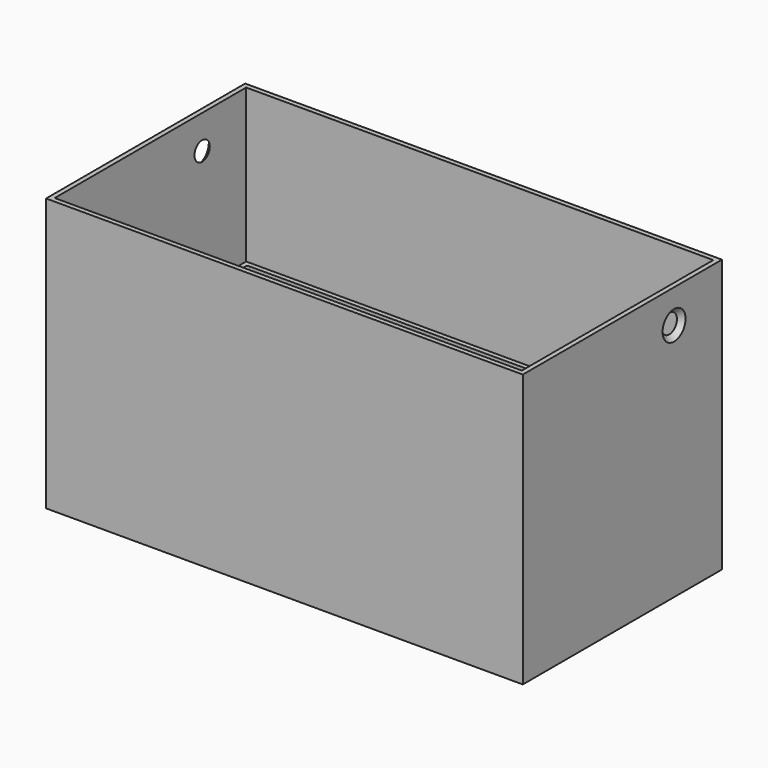
from build123d import *

# Parameters (mm, degrees)
F1_W          = 95.6
F1_H          = 48
F1_R          = 3
F1_R_2        = 1.75
F2_DEPTH      = 1.5
F1_W_2        = 97.6
F1_H_2        = 50
F3_DEPTH      = 25
F1_W_3        = 99.6
F1_H_3        = 52
F4_DEPTH      = 57
F5_R          = 2
F6_DEPTH      = 49.801
F6_DEPTH_BACK = 49.801
F7_SIZE       = 0.99999
F8_R          = 0.5


# Not quite as in the source:
# - a fillet or chamfer is up to 0.001 mm smaller than in the source, because OpenCascade refuses the exact size


with BuildPart() as f2:
    # F1 (on Top) → F2 (new body)
    with BuildSketch(Plane.XY):
        Rectangle(F1_W, F1_H)
        with Locations((-34.0166666667, 0)):
            Circle(F1_R, mode=Mode.SUBTRACT)
        with Locations((-20.2333333333, 0)):
            Circle(F1_R, mode=Mode.SUBTRACT)
        with Locations((-6.45, 0)):
            Circle(F1_R_2, mode=Mode.SUBTRACT)
        Polygon((-2.2, -13.3), (-2.2, 13.3), (35, 13.3), (40.3, 8), (40.3, -8), (35, -13.3), align=None, mode=Mode.SUBTRACT)
        with Locations((44.55, 0)):
            Circle(F1_R_2, mode=Mode.SUBTRACT)
    extrude(amount=F2_DEPTH)

    # F1 (on Top) → F3 (join)
    with BuildSketch(Plane.XY):
        Rectangle(F1_W_2, F1_H_2)
        Rectangle(F1_W, F1_H, mode=Mode.SUBTRACT)
    extrude(amount=F3_DEPTH)

    # F1 (on Top) → F4 (join)
    with BuildSketch(Plane.XY):
        Rectangle(F1_W_3, F1_H_3)
        Rectangle(F1_W_2, F1_H_2, mode=Mode.SUBTRACT)
    extrude(amount=F4_DEPTH)

    # F5 (on Right) → F6 (cut, two sides)
    with BuildSketch(Plane.YZ) as f6_sk:
        with Locations((13.5, 50)):
            Circle(F5_R)
    extrude(amount=-F6_DEPTH, mode=Mode.SUBTRACT)
    extrude(f6_sk.sketch, amount=F6_DEPTH_BACK, mode=Mode.SUBTRACT)

    # F7 (size 1 in the source; OpenCascade refuses exactly that, so slightly less here)
    f7_edges = [f2.edges().sort_by_distance(p)[0] for p in [
        (49.8, 11.5, 50),
        (-49.8, 11.5, 50),
    ]]
    chamfer(f7_edges, length=F7_SIZE)

    # F8
    f8_edges = [f2.edges().sort_by_distance(p)[0] for p in [
        (-17.233333, 0, 0.75),
        (-23.233333, 0, 0),
        (-23.233333, 0, 1.5),
        (-31.016667, 0, 0.75),
        (-37.016667, 0, 0),
        (-37.016667, 0, 1.5),
        (-47.8, 0, 1.5),
        (0, 24, 1.5),
        (47.8, 0, 1.5),
        (47.8, 24, 13.25),
        (-47.8, 24, 13.25),
        (-47.8, -24, 13.25),
        (0, -24, 1.5),
        (47.8, -24, 13.25),
    ]]
    fillet(f8_edges, radius=F8_R)


solid = f2.part
